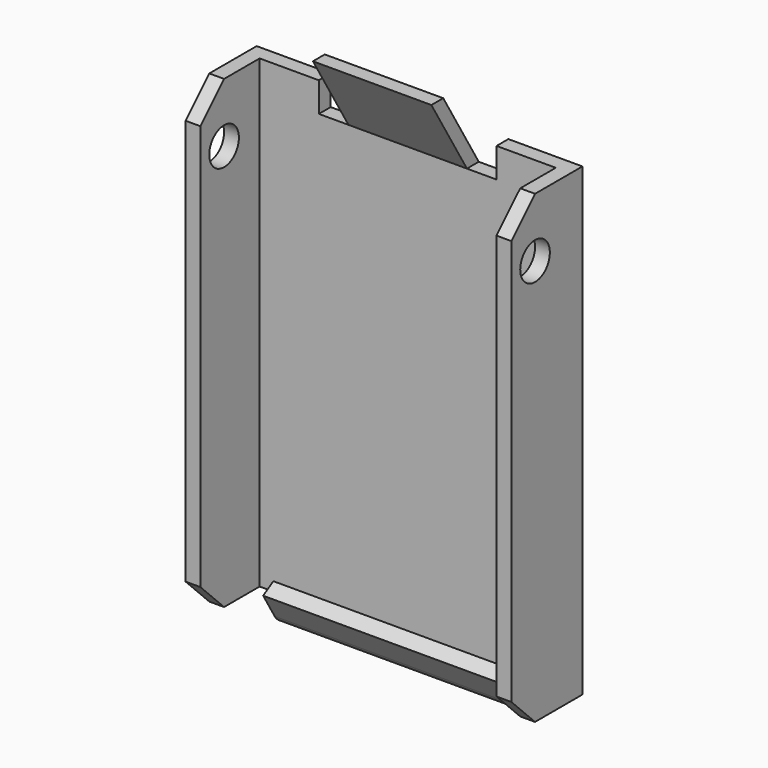
from build123d import *

# Parameters (mm, degrees)
F1_DEPTH  = 3.175
F3_DEPTH  = 3.175
F6_W      = 50.8
F6_H      = 3.175
F9_W      = 25.4
F9_H      = 3.175
F12_R     = 3.96875
F13_DEPTH = 69.851


# Not quite as in the source:
# - a feature of the source that left no trace in its solid (it failed there, or was rolled back) is left out
# - a pattern or mirror of a feature is missing from the dataset's text; its kind, count and spacing are read off the source's solid


with BuildPart() as f1:
    # F0 (on Front) → F1 (new body)
    with BuildSketch(Plane.XZ):
        Polygon((0, 99.695), (0, 0), (63.5, 0), (63.5, 99.695), (50.8, 99.695), (50.8, 93.345), (12.7, 93.345), (12.7, 99.695), align=None)
    extrude(amount=F1_DEPTH)

    # F2 (on Right) → F3 (join)
    with BuildSketch(Plane.YZ):
        Polygon((-12.7, 0), (0, 0), (0, 99.695), (-12.7, 99.695), (-19.05, 93.345), (-19.05, 6.35), align=None)
    f3 = extrude(amount=-F3_DEPTH)

    # F3_copies: F3 across plane
    add(f3.mirror(Plane(origin=(31.75, 0, 0), x_dir=(0, 0, 1), z_dir=(1, 0, 0))))

    # F8: sweep along a path in F7
    with BuildLine(Plane.YZ) as f8_path:
        ThreePointArc((0, 0), (-2.7925061525, -3.6716217493), (-7.0765387245, -1.9610774491))
        Line((-7.0765387245, -1.9610774491), (-10.16, 3.175))
    # F6 (on face) → F8 (sweep)
    with BuildSketch(Plane(origin=(0, 0, 0), x_dir=(1, 0, 0), z_dir=(0, 0, -1))):
        with Locations((31.75, 1.5875)):
            Rectangle(F6_W, F6_H)
    sweep(path=f8_path.line)

    # F11: sweep along a path in F10
    with BuildLine(Plane.YZ) as f11_path:
        Line((-3.175, 93.345), (-12.7, 109.22))
    # F9 (on face) → F11 (sweep)
    with BuildSketch(Plane.XY.offset(93.345)):
        with Locations((31.75, -1.5875)):
            Rectangle(F9_W, F9_H)
    sweep(path=f11_path.line)

    # F12 (on face) → F13 (cut, through all)
    with BuildSketch(Plane(origin=(-3.175, 0, 0), x_dir=(0, -1, 0), z_dir=(-1, 0, 0))):
        with Locations((12.7, 86.995)):
            Circle(F12_R)
    extrude(amount=-F13_DEPTH, mode=Mode.SUBTRACT)


solid = f1.part
